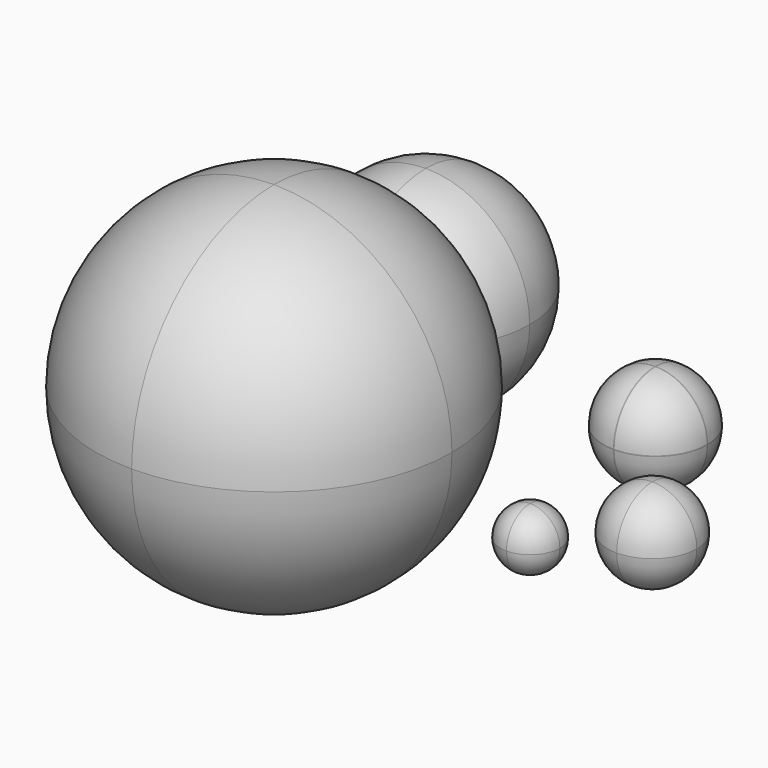
from build123d import *

# Parameters (mm, degrees)
F0_W      = 60
F0_H      = 60
F1_DEPTH  = 60
F2_R      = 29.99999
F3_W      = 10
F3_H      = 10
F4_DEPTH  = 10
F5_R      = 4.99999
F6_W      = 15
F6_H      = 15
F7_DEPTH  = 15
F8_R      = 7.49999
F9_W      = 17.5
F9_H      = 17.5
F10_DEPTH = 17.5
F11_R     = 8.7
F12_W     = 35
F12_H     = 35
F13_DEPTH = 35
F14_R     = 17.49999
F15_W     = 10
F15_H     = 10
F16_DEPTH = 10
F17_R     = 4.99999


# Not quite as in the source:
# - a fillet or chamfer is up to 0.001 mm smaller than in the source, because OpenCascade refuses the exact size


with BuildPart() as f1:
    # F0 (on Top) → F1 (new body)
    with BuildSketch(Plane.XY):
        Rectangle(F0_W, F0_H)
    extrude(amount=F1_DEPTH)

    # F2 (radius 30 in the source; OpenCascade refuses exactly that, so slightly less here)
    f2_edges = [f1.edges().sort_by_distance(p)[0] for p in [
        (30, -30, 30),
        (-30, -30, 30),
        (0, -30, 0),
        (0, -30, 60),
        (0, 30, 0),
        (-30, 0, 0),
        (30, 0, 0),
        (30, 30, 30),
        (30, 0, 60),
        (-30, 30, 30),
        (0, 30, 60),
        (-30, 0, 60),
    ]]
    fillet(f2_edges, radius=F2_R)


with BuildPart() as f4:
    # F3 (on Top) → F4 (new body)
    with BuildSketch(Plane.XY):
        with Locations((23.1205523014, 25.0656651421)):
            Rectangle(F3_W, F3_H)
    extrude(amount=F4_DEPTH)

    # F5 (radius 5 in the source; OpenCascade refuses exactly that, so slightly less here)
    f5_edges = [f4.edges().sort_by_distance(p)[0] for p in [
        (28.120552, 30.065665, 5),
        (18.120552, 20.065665, 5),
        (28.120552, 25.065665, 0),
        (28.120552, 25.065665, 10),
        (23.120552, 20.065665, 10),
        (23.120552, 20.065665, 0),
        (28.120552, 20.065665, 5),
        (23.120552, 30.065665, 0),
        (18.120552, 25.065665, 0),
        (18.120552, 30.065665, 5),
        (23.120552, 30.065665, 10),
        (18.120552, 25.065665, 10),
    ]]
    fillet(f5_edges, radius=F5_R)


with BuildPart() as f7:
    # F6 (on Top) → F7 (new body)
    with BuildSketch(Plane.XY):
        with Locations((37.8113878518, 32.4358163551)):
            Rectangle(F6_W, F6_H)
    extrude(amount=F7_DEPTH)

    # F8 (radius 7.5 in the source; OpenCascade refuses exactly that, so slightly less here)
    f8_edges = [f7.edges().sort_by_distance(p)[0] for p in [
        (45.311388, 24.935816, 7.5),
        (45.311388, 39.935816, 7.5),
        (45.311388, 32.435816, 0),
        (45.311388, 32.435816, 15),
        (37.811388, 39.935816, 15),
        (30.311388, 39.935816, 7.5),
        (37.811388, 39.935816, 0),
        (30.311388, 24.935816, 7.5),
        (37.811388, 24.935816, 15),
        (37.811388, 24.935816, 0),
        (30.311388, 32.435816, 0),
        (30.311388, 32.435816, 15),
    ]]
    fillet(f8_edges, radius=F8_R)


with BuildPart() as f10:
    # F9 (on Top) → F10 (new body)
    with BuildSketch(Plane.XY):
        with Locations((20.5947593786, 54.6041680584)):
            Rectangle(F9_W, F9_H)
    extrude(amount=F10_DEPTH)

    # F11
    f11_edges = [f10.edges().sort_by_distance(p)[0] for p in [
        (11.844759, 54.604168, 0),
        (20.594759, 63.354168, 0),
        (11.844759, 45.854168, 8.75),
        (29.344759, 63.354168, 8.75),
        (29.344759, 54.604168, 17.5),
        (20.594759, 45.854168, 17.5),
        (11.844759, 63.354168, 8.75),
        (11.844759, 54.604168, 17.5),
        (29.344759, 45.854168, 8.75),
        (20.594759, 45.854168, 0),
        (20.594759, 63.354168, 17.5),
        (29.344759, 54.604168, 0),
    ]]
    fillet(f11_edges, radius=F11_R)


with BuildPart() as f13:
    # F12 (on Top) → F13 (new body)
    with BuildSketch(Plane.XY):
        with Locations((-17.2741941642, 53.5828206353)):
            Rectangle(F12_W, F12_H)
    extrude(amount=F13_DEPTH)

    # F14 (radius 17.5 in the source; OpenCascade refuses exactly that, so slightly less here)
    f14_edges = [f13.edges().sort_by_distance(p)[0] for p in [
        (0.225806, 53.582821, 35),
        (0.225806, 36.082821, 17.5),
        (0.225806, 71.082821, 17.5),
        (0.225806, 53.582821, 0),
        (-17.274194, 71.082821, 35),
        (-34.774194, 36.082821, 17.5),
        (-17.274194, 36.082821, 0),
        (-17.274194, 36.082821, 35),
        (-34.774194, 53.582821, 35),
        (-17.274194, 71.082821, 0),
        (-34.774194, 53.582821, 0),
        (-34.774194, 71.082821, 17.5),
    ]]
    fillet(f14_edges, radius=F14_R)


with BuildPart() as f16:
    # F15 (on Top) → F16 (new body)
    with BuildSketch(Plane.XY):
        with Locations((-45.0907275081, 56.3959827726)):
            Rectangle(F15_W, F15_H)
    extrude(amount=F16_DEPTH)

    # F17 (radius 5 in the source; OpenCascade refuses exactly that, so slightly less here)
    f17_edges = [f16.edges().sort_by_distance(p)[0] for p in [
        (-45.090728, 61.395983, 10),
        (-50.090728, 56.395983, 10),
        (-45.090728, 51.395983, 10),
        (-40.090728, 56.395983, 10),
        (-50.090728, 51.395983, 5),
        (-45.090728, 61.395983, 0),
        (-50.090728, 56.395983, 0),
        (-45.090728, 51.395983, 0),
        (-40.090728, 56.395983, 0),
        (-40.090728, 61.395983, 5),
        (-50.090728, 61.395983, 5),
        (-40.090728, 51.395983, 5),
    ]]
    fillet(f17_edges, radius=F17_R)


solid = Compound([f1.part, f4.part, f7.part, f10.part, f13.part, f16.part])
